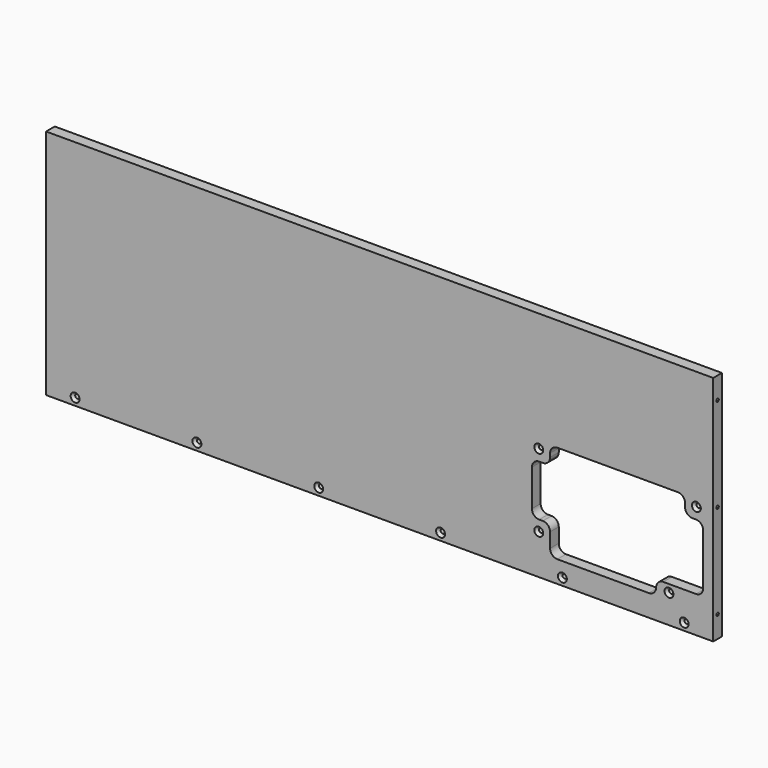
from build123d import *

# Parameters (mm, degrees)
F0_W           = 584.2
F0_H           = 203.2
F1_DEPTH       = 9.525
F3_D           = 3.6576
F3_DEPTH       = 10.3124
F3_CSINK_D     = 7.7978
F3_CSINK_ANGLE = 82
F3_TIP         = 1.0988539001
F4_W           = 101.6
F4_H           = 69.85
F5_DEPTH       = 9.526
F6_DEPTH       = 25.4
F9_D           = 2.7051
F9_DEPTH       = 13.4874
F9_TIP         = 0.8126940303
F9_ON_F7_D     = 2.7051
F9_ON_F7_DEPTH = 13.4874
F9_ON_F7_TIP   = 0.8126940303


# Not quite as in the source:
# - a feature names something its author has since deleted; it is built from what else it names


with BuildPart() as f1:
    # F0 (on Front) → F1 (new body)
    with BuildSketch(Plane.XZ):
        with Locations((-292.1, 101.6)):
            Rectangle(F0_W, F0_H)
    extrude(amount=F1_DEPTH)

    # F3
    with Locations(Plane.XZ.offset(9.525)):
        with Locations((-238.76, 6.35), (-25.4, 6.35), (-345.44, 6.35), (-558.8, 6.35), (-132.08, 6.35), (-452.12, 6.35), (-152.75, 99.05), (-152.75, 35.05), (-38.75, 25.05), (-14.75, 99.05)):
            CounterSinkHole(F3_D / 2, F3_CSINK_D / 2, depth=F3_DEPTH, counter_sink_angle=F3_CSINK_ANGLE)
            with Locations((0, 0, -(F3_DEPTH + F3_TIP / 2))):  # 118° drill point
                Cone(0, F3_D / 2, F3_TIP, mode=Mode.SUBTRACT)

    # F4 (on face) → F5 (cut, through all)
    with BuildSketch(Plane.XZ.offset(9.525)):
        with Locations((-76.2, 66.675)):
            Rectangle(F4_W, F4_H)
    extrude(amount=-F5_DEPTH, mode=Mode.SUBTRACT)

    # F2 (on face) → F6 (cut)
    with BuildSketch(Plane.XZ.offset(9.525)):
        with BuildLine():
            Line((-30.975, 105.05), (-136.525, 105.05))
            ThreePointArc((-136.525, 105.05), (-141.0151280605, 103.1901280605), (-142.875, 98.7))
            Line((-142.875, 98.7), (-142.875, 95.525))
            ThreePointArc((-142.875, 95.525), (-144.7348719395, 91.0348719395), (-149.225, 89.175))
            Line((-149.225, 89.175), (-152.4, 89.175))
            ThreePointArc((-152.4, 89.175), (-156.8901280605, 87.3151280605), (-158.75, 82.825))
            Line((-158.75, 82.825), (-158.75, 50.8))
            ThreePointArc((-158.75, 50.8), (-156.8901280605, 46.3098719395), (-152.4, 44.45))
            Line((-152.4, 44.45), (-149.225, 44.45))
            ThreePointArc((-149.225, 44.45), (-144.7348719395, 42.5901280605), (-142.875, 38.1))
            Line((-142.875, 38.1), (-142.875, 25.4))
            ThreePointArc((-142.875, 25.4), (-141.0151280605, 20.9098719395), (-136.525, 19.05))
            Line((-136.525, 19.05), (-56.375, 19.05))
            ThreePointArc((-56.375, 19.05), (-51.8848719395, 20.9098719395), (-50.025, 25.4))
            ThreePointArc((-50.025, 25.4), (-48.1651280605, 29.8901280605), (-43.675, 31.75))
            Line((-43.675, 31.75), (-15.1, 31.75))
            ThreePointArc((-15.1, 31.75), (-10.6098719395, 33.6098719395), (-8.75, 38.1))
            Line((-8.75, 38.1), (-8.75, 82.825))
            ThreePointArc((-8.75, 82.825), (-10.6098719395, 87.3151280605), (-15.1, 89.175))
            Line((-15.1, 89.175), (-18.275, 89.175))
            ThreePointArc((-18.275, 89.175), (-22.7651280605, 91.0348719395), (-24.625, 95.525))
            Line((-24.625, 95.525), (-24.625, 98.7))
            ThreePointArc((-24.625, 98.7), (-26.4848719395, 103.1901280605), (-30.975, 105.05))
        make_face()
    extrude(amount=-F6_DEPTH, mode=Mode.SUBTRACT)

    # F9
    with Locations(Plane.YZ):
        with Locations((-4.7625, 184.15), (-4.7625, 101.6), (-4.7625, 19.05)):
            Hole(F9_D / 2, depth=F9_DEPTH)
            with Locations((0, 0, -(F9_DEPTH + F9_TIP / 2))):  # 118° drill point
                Cone(0, F9_D / 2, F9_TIP, mode=Mode.SUBTRACT)

    # F9 on F7
    with Locations(Plane(origin=(-584.2, 0, 0), x_dir=(0, -1, 0), z_dir=(-1, 0, 0))):
        with Locations((4.7625, 184.15), (4.7625, 101.6), (4.7625, 19.05)):
            Hole(F9_ON_F7_D / 2, depth=F9_ON_F7_DEPTH)
            with Locations((0, 0, -(F9_ON_F7_DEPTH + F9_ON_F7_TIP / 2))):  # 118° drill point
                Cone(0, F9_ON_F7_D / 2, F9_ON_F7_TIP, mode=Mode.SUBTRACT)


solid = f1.part
